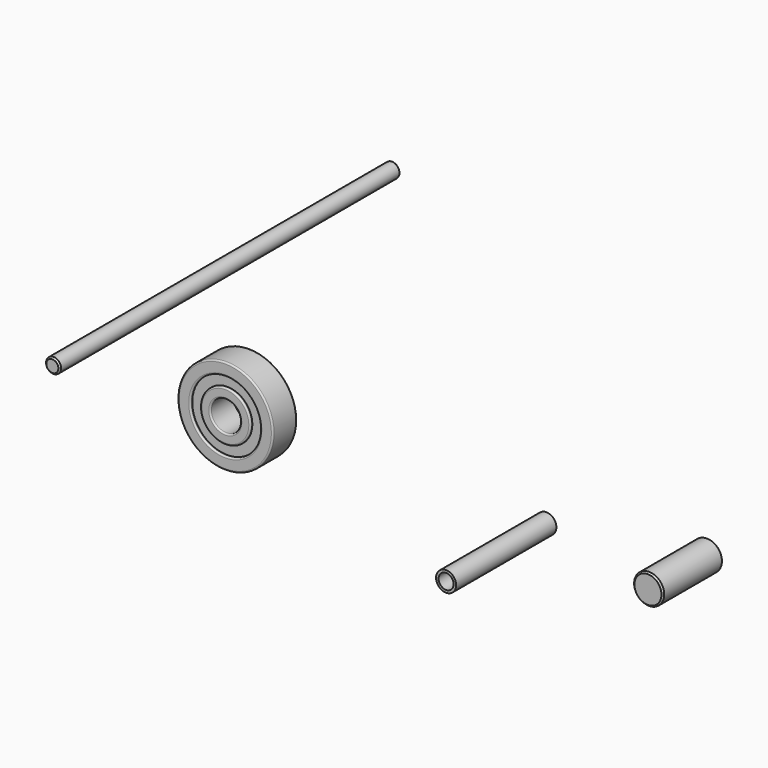
from build123d import *

# Parameters (mm, degrees)
F0_R      = 3
F1_DEPTH  = 7.5
F2_SIZE   = 0.3
F3_R      = 2
F3_R_2    = 1.5
F4_DEPTH  = 25
F5_R      = 9.5
F5_R_2    = 3
F6_DEPTH  = 3
F7_R      = 0.3
F8_R      = 7
F8_R_2    = 5
F9_DEPTH  = 0.5
F10_R     = 0.3
F11_R     = 1.5
F12_DEPTH = 85
F13_SIZE  = 0.3


# Not quite as in the source:
# - a pattern or mirror of a feature is missing from the dataset's text; its kind, count and spacing are read off the source's solid


with BuildPart() as f1:
    # F0 (on Front) → F1 (new body, symmetric)
    with BuildSketch(Plane.XZ):
        with Locations((56.8486019969, 0)):
            Circle(F0_R)
    extrude(amount=F1_DEPTH, both=True)

    # F2
    f2_edges = [f1.edges().sort_by_distance(p)[0] for p in [
        (53.848602, -7.5, 0),
        (53.848602, 7.5, 0),
    ]]
    chamfer(f2_edges, length=F2_SIZE)


with BuildPart() as f4:
    # F3 (on Front) → F4 (new body)
    with BuildSketch(Plane.XZ):
        with Locations((30.5693875998, 0)):
            Circle(F3_R)
        with Locations((30.5693875998, 0)):
            Circle(F3_R_2, mode=Mode.SUBTRACT)
    extrude(amount=F4_DEPTH)


with BuildPart() as f6:
    # F5 (on Front) → F6 (new body, symmetric)
    with BuildSketch(Plane.XZ):
        with Locations((-31.095571816, 0)):
            Circle(F5_R)
        with Locations((-31.095571816, 0)):
            Circle(F5_R_2, mode=Mode.SUBTRACT)
    extrude(amount=F6_DEPTH, both=True)

    # F7
    f7_edges = [f6.edges().sort_by_distance(p)[0] for p in [
        (-40.595572, -3, 0),
        (-34.095572, -3, 0),
        (-34.095572, 3, 0),
        (-40.595572, 3, 0),
    ]]
    fillet(f7_edges, radius=F7_R)

    # F8 (on face) → F9 (cut)
    with BuildSketch(Plane.XZ.offset(3)):
        with Locations((-31.095571816, 0)):
            Circle(F8_R)
        with Locations((-31.095571816, 0)):
            Circle(F8_R_2, mode=Mode.SUBTRACT)
    f9 = extrude(amount=-F9_DEPTH, mode=Mode.SUBTRACT)

    # F9_copies: F9 across plane
    add(f9.mirror(Plane.ZX), mode=Mode.SUBTRACT)

    # F10
    f10_edges = [f6.edges().sort_by_distance(p)[0] for p in [
        (-34.395572, -3, 0),
        (-36.095572, -3, 0),
        (-38.095572, -3, 0),
        (-38.095572, 3, 0),
        (-36.095572, 3, 0),
    ]]
    fillet(f10_edges, radius=F10_R)


with BuildPart() as f12:
    # F11 (on Front) → F12 (new body)
    with BuildSketch(Plane.XZ):
        with Locations((0, 19.2675273865)):
            Circle(F11_R)
    extrude(amount=F12_DEPTH)

    # F13
    f13_edges = [f12.edges().sort_by_distance(p)[0] for p in [
        (-1.5, -85, 19.267527),
        (-1.5, 0, 19.267527),
    ]]
    chamfer(f13_edges, length=F13_SIZE)


with BuildPart() as f12_1:
    # F14: moved
    add(f12.part.moved(Location((0, 0, 33))))


solid = Compound([f1.part, f4.part, f6.part, f12_1.part])
